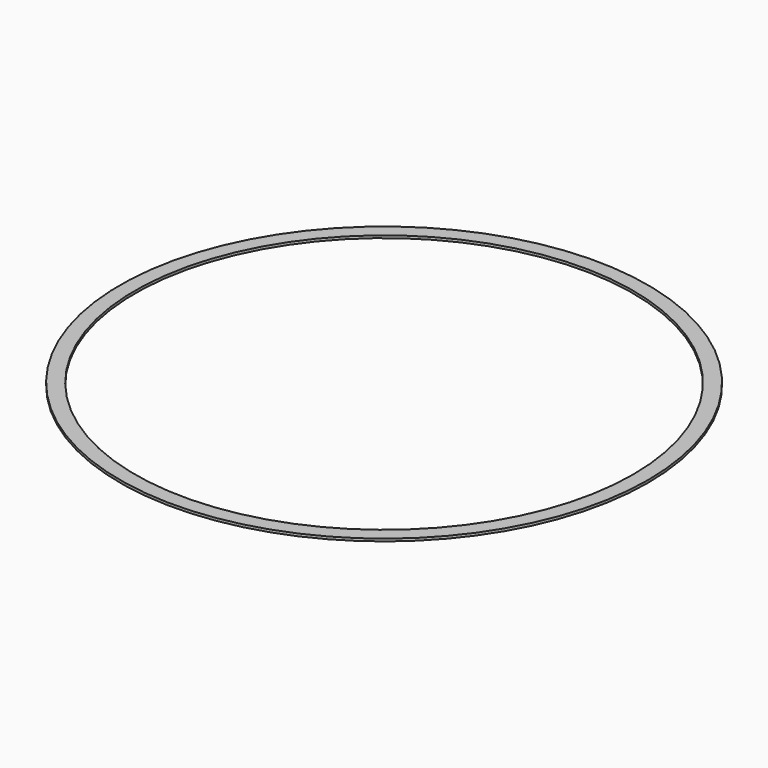
from build123d import *

# Parameters (mm, degrees)
F0_R     = 448.73926
F0_R_2   = 423.33926
F1_DEPTH = 4.2333333333


# Not quite as in the source:
# - a length typed as a fraction of an inch, garbled in the dataset ("3 / 203.2 mm" for 3/8 in), is restored


with BuildPart() as f1:
    # F0 (on Top) → F1 (new body)
    with BuildSketch(Plane.XY):
        Circle(F0_R)
        Circle(F0_R_2, mode=Mode.SUBTRACT)
    extrude(amount=F1_DEPTH)


solid = f1.part
